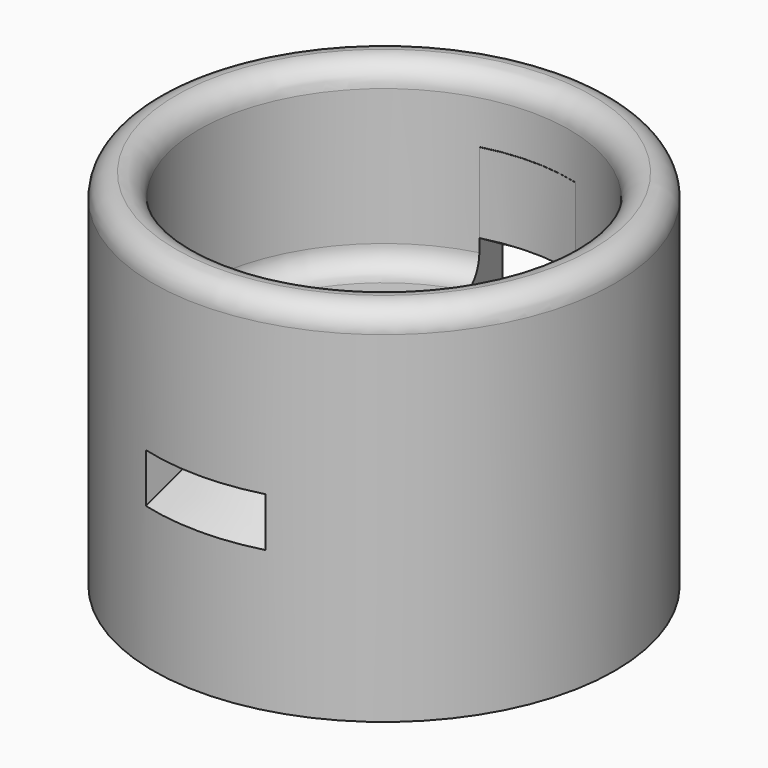
from build123d import *

# Parameters (mm, degrees)
F1_R          = 16.129
F2_DEPTH      = 25.4
F3_R          = 12.954
F4_DEPTH      = 12.7
F5_R          = 1.58749
F7_ANGLE_BACK = 15
F7_ANGLE      = 30
F8_T4_ANGLE   = 47.2856392703
F8_S5_R       = 12.954
F8_T6_DEPTH   = 7
F8_T10_ANGLE  = 47.2856392703
F8_S11_R      = 12.954
F8_T12_DEPTH  = 7


# Not quite as in the source:
# - a fillet or chamfer that OpenCascade refuses, or shapes differently, is made with other operations: its cross-section is extruded or revolved along the edge and cut away or added
# - a fillet or chamfer is up to 0.001 mm smaller than in the source, because OpenCascade refuses the exact size
# - ends of sketch curves that miss each other by under 0.0002 mm in the source are joined


with BuildPart() as f2:
    # F1 (on Top) → F2 (new body)
    with BuildSketch(Plane.XY):
        Circle(F1_R)
    extrude(amount=F2_DEPTH)

    # F3 (on face) → F4 (cut)
    with BuildSketch(Plane.XY.offset(25.4)):
        Circle(F3_R)
    extrude(amount=-F4_DEPTH, mode=Mode.SUBTRACT)

    # F5 (radius 1.5875 in the source; OpenCascade refuses exactly that, so slightly less here)
    f5_edges = [f2.edges().sort_by_distance(p)[0] for p in [
        (-16.129, 0, 25.4),
        (-12.954, 0, 25.4),
        (-12.954, 0, 12.7),
    ]]
    fillet(f5_edges, radius=F5_R)

    # F6 (on Right) → F7 (revolve, cut)
    with BuildSketch(Plane.YZ, mode=Mode.PRIVATE) as f7_sk:
        with BuildLine():
            ThreePointArc((12.2294899884, 15.6199430682), (12.8889010018, 13.8375539592), (11.3665, 12.7))
            Line((11.3665, 12.7), (16.129, 9.8708188202))
            Line((16.129, 9.8708188202), (16.129, 13.3034244871))
            Line((16.129, 13.3034244871), (12.9914900466, 15.1672741693))
            Line((12.9914900466, 15.1672741693), (12.2294899884, 15.6199430682))
        make_face()
        with BuildLine():
            Line((-16.129, 9.8708188202), (-11.3665, 12.7))
            ThreePointArc((-11.3665, 12.7), (-12.8889010018, 13.8375539592), (-12.2294899884, 15.6199430682))
            Line((-12.2294899884, 15.6199430682), (-12.9914900466, 15.1672741693))
            Line((-12.9914900466, 15.1672741693), (-16.129, 13.3034244871))
            Line((-16.129, 13.3034244871), (-16.129, 9.8708188202))
        make_face()
        Polygon((12.2294900466, 21.5172741693), (12.2294900466, 15.6199431581), (12.9914900466, 15.1672741693), (12.9914900466, 21.5172741693), align=None)
        Polygon((-12.9914900466, 15.1672741693), (-12.2294900466, 15.6199431581), (-12.2294900466, 21.5172741693), (-12.9914900466, 21.5172741693), align=None)
    revolve(f7_sk.sketch.rotate(Axis((0, 0, 7.0286970586), (0, 0, -1)), -F7_ANGLE_BACK), axis=Axis((0, 0, 7.0286970586), (0, 0, -1)), revolution_arc=F7_ANGLE, mode=Mode.SUBTRACT)

    # F8: chamfer of 0.762 on 2 edges, made by hand


with BuildPart() as f8_tool2:
    # F8_s3 → F8_t4 (revolve)
    with BuildSketch(Plane(origin=(0, 0, 0), x_dir=(0, 0, 1), z_dir=(0.9160632754, 0.4010337585, 0))):
        Polygon((21.5172741693, 12.2294900466), (20.7552741693, 12.9914900466), (21.5172741693, 12.9914900466), align=None)
    revolve(axis=Axis((0, 0, 21.5172741693), (0, 0, -1)), revolution_arc=F8_T4_ANGLE)

    # F8_s5 → F8_t6 (cut, symmetric)
    with BuildSketch(Plane.XY.offset(21.1)):
        Circle(F8_S5_R)
    extrude(amount=F8_T6_DEPTH, both=True, mode=Mode.SUBTRACT)


with BuildPart() as f2_1:
    add(f2.part)

    # F8_t1: union F8_tool2
    add(f8_tool2.part)


with BuildPart() as f8_tool8:
    # F8_s9 → F8_t10 (revolve)
    with BuildSketch(Plane(origin=(0, 0, 0), x_dir=(0, 0, 1), z_dir=(-0.9160632754, -0.4010337585, 0))):
        Polygon((21.5172741693, 12.2294900466), (20.7552741693, 12.9914900466), (21.5172741693, 12.9914900466), align=None)
    revolve(axis=Axis((0, 0, 21.5172741693), (0, 0, -1)), revolution_arc=F8_T10_ANGLE)

    # F8_s11 → F8_t12 (cut, symmetric)
    with BuildSketch(Plane.XY.offset(21.1)):
        Circle(F8_S11_R)
    extrude(amount=F8_T12_DEPTH, both=True, mode=Mode.SUBTRACT)


with BuildPart() as f2_2:
    add(f2_1.part)

    # F8_t7: union F8_tool8
    add(f8_tool8.part)


solid = f2_2.part
